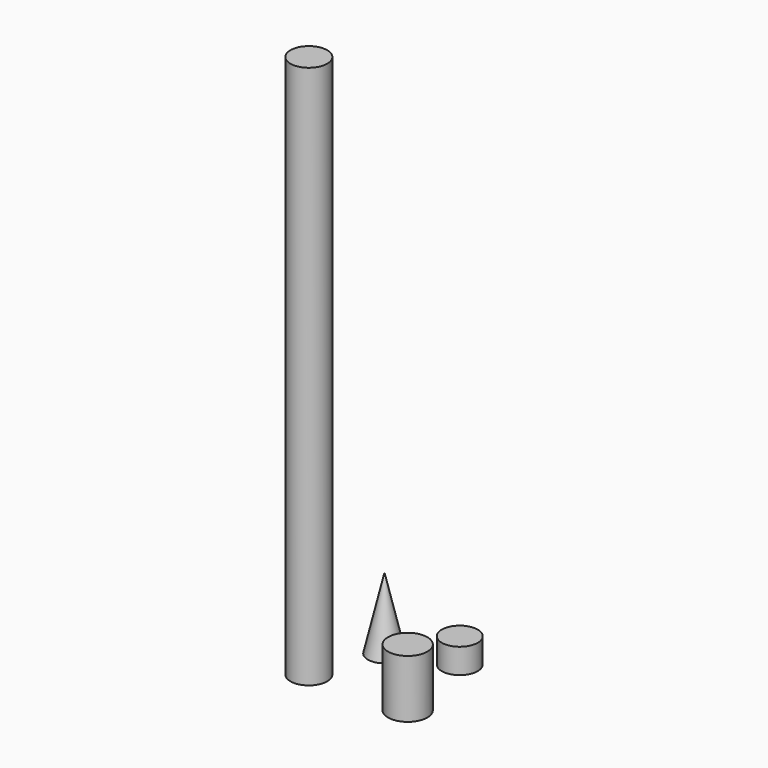
from build123d import *

# Parameters (mm, degrees)
F0_R     = 19.9680226168
F1_DEPTH = 59.0213239193
F2_R     = 18.2371893678
F3_DEPTH = 25.4
F6_R     = 18.6649469358
F7_DEPTH = 552.8296232224
F8_R     = 17.8826234865
F9_DEPTH = 72.1546784043


# Not quite as in the source:
# - a fillet or chamfer that OpenCascade refuses, or shapes differently, is made with other operations: its cross-section is extruded or revolved along the edge and cut away or added
# - the program builds the solid bodies; features that only make, move or delete a surface that nothing else refers to are left out


with BuildPart() as f1:
    # F0 (on Top) → F1 (new body)
    with BuildSketch(Plane.XY):
        with Locations((52.6638887823, -46.1734086275)):
            Circle(F0_R)
    extrude(amount=F1_DEPTH)


with BuildPart() as f3:
    # F2 (on Top) → F3 (new body)
    with BuildSketch(Plane.XY):
        with Locations((35.7855930924, 41.0611107945)):
            Circle(F2_R)
    extrude(amount=F3_DEPTH)


with BuildPart() as f7:
    # F6 (on Top) → F7 (new body)
    with BuildSketch(Plane.XY):
        with Locations((-46.9713956118, -47.2776144743)):
            Circle(F6_R)
    extrude(amount=F7_DEPTH)


with BuildPart() as f9:
    # F8 (on Top) → F9 (new body)
    with BuildSketch(Plane.XY):
        with Locations((-22.7211695164, 18.5588113964)):
            Circle(F8_R)
    extrude(amount=F9_DEPTH)

    # F10: chamfer of 17.78 x 76.2 on 1 edges, made by hand

    # F10_s1 → F10_t2 (revolve, cut)
    with BuildSketch(Plane.XZ.offset(-18.5588113964)):
        Polygon((-4.8385460299, -4.0453215957), (-22.6185460299, 72.1546784043), (-4.8385460299, 72.1546784043), align=None)
    revolve(axis=Axis((-22.7211695164, 18.5588113964, 72.1546784043), (0, 0, 1)), mode=Mode.SUBTRACT)


solid = Compound([f1.part, f3.part, f7.part, f9.part])
